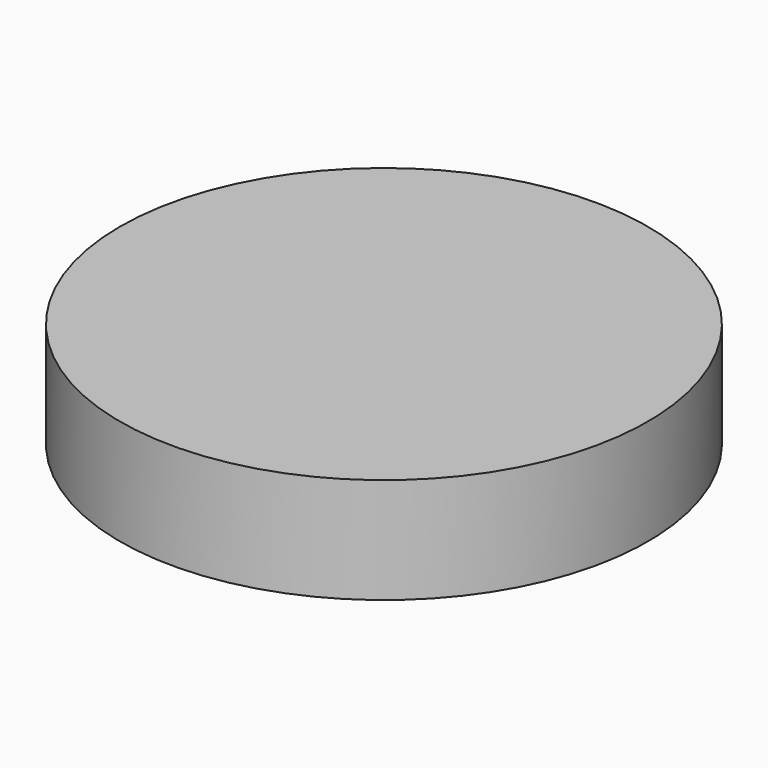
from build123d import *

# Parameters (mm, degrees)
F0_W = 37.5
F0_H = 7.5
F2_T = -0.5


# Not quite as in the source:
# - a feature names something its author has since deleted; it is built from what else it names


with BuildPart() as f1:
    # F0 (on Front) → F1 (revolve)
    with BuildSketch(Plane.XZ):
        with Locations((-18.75, -3.75)):
            Rectangle(F0_W, F0_H)
        with Locations((-18.75, 3.75)):
            Rectangle(F0_W, F0_H)
    revolve(axis=Axis((0, 0, -0.1110713929), (0, 0, -1)))

    # F2
    f2_openings = [f1.faces().sort_by_distance(p)[0] for p in [
        (0, 0, -7.5),
    ]]
    offset(amount=F2_T, openings=f2_openings)


solid = f1.part
